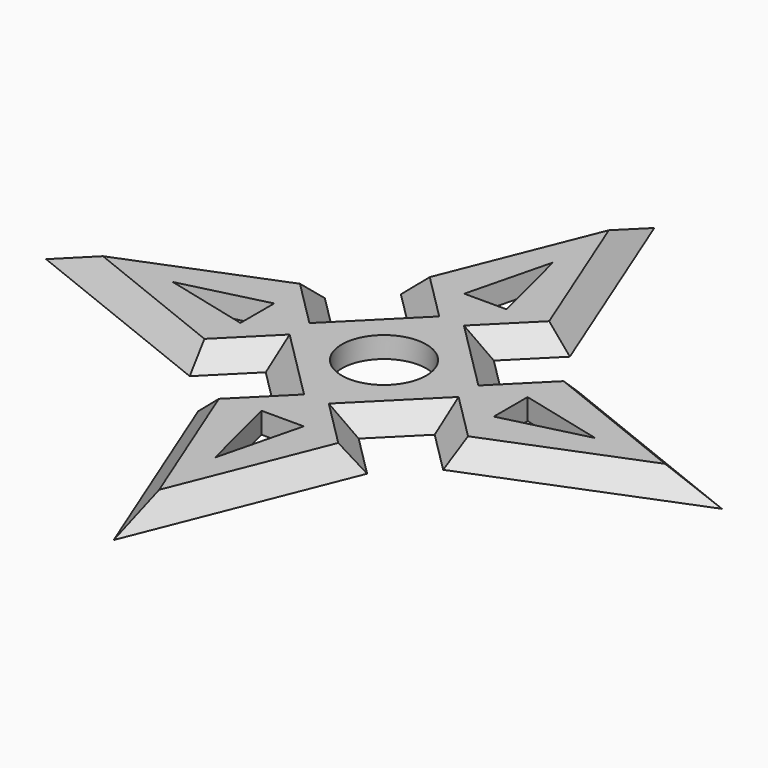
from build123d import *

# Parameters (mm, degrees)
F0_R     = 6.35
F1_DEPTH = 3.175
F2_SIZE  = 3.17499


# Not quite as in the source:
# - a fillet or chamfer is up to 0.001 mm smaller than in the source, because OpenCascade refuses the exact size


with BuildPart() as f1:
    # F0 (on Top) → F1 (new body)
    with BuildSketch(Plane.XY):
        Polygon((6.35, -12.6999929847), (-6.35, -12.6999929847), (-12.6999929847, -19.0499859695), (0, -50.7999929847), (12.6999929847, -19.0499859695), align=None)
        Polygon((-3.175, -19.0499929847), (3.175, -19.0499929847), (0, -31.7499929847), align=None, mode=Mode.SUBTRACT)
        Polygon((19.0499859695, 12.6999929847), (12.6999929847, 6.35), (12.6999929847, -6.35), (19.0499859695, -12.6999929847), (50.7999929847, 0), align=None)
        Polygon((19.0499929847, -3.175), (19.0499929847, 3.175), (31.7499929847, 0), align=None, mode=Mode.SUBTRACT)
        Polygon((-6.35, 12.6999929847), (-12.6999929847, 6.35), (-12.6999929847, -6.35), (-6.35, -12.6999929847), (6.35, -12.6999929847), (12.6999929847, -6.35), (12.6999929847, 6.35), (6.35, 12.6999929847), align=None)
        Circle(F0_R, mode=Mode.SUBTRACT)
        Polygon((-12.6999929847, -6.35), (-12.6999929847, 6.35), (-19.0499859695, 12.6999929847), (-50.7999929847, 0), (-19.0499859695, -12.6999929847), align=None)
        Polygon((-19.0499929847, 3.175), (-19.0499929847, -3.175), (-31.7499929847, 0), align=None, mode=Mode.SUBTRACT)
        Polygon((-12.6999929847, 19.0499859695), (-6.35, 12.6999929847), (6.35, 12.6999929847), (12.6999929847, 19.0499859695), (0, 50.7999929847), align=None)
        Polygon((3.175, 19.0499929847), (-3.175, 19.0499929847), (0, 31.7499929847), align=None, mode=Mode.SUBTRACT)
    extrude(amount=F1_DEPTH)

    # F2 (size 3.175 in the source; OpenCascade refuses exactly that, so slightly less here)
    f2_edges = [f1.edges().sort_by_distance(p)[0] for p in [
        (6.349996, -34.924989, 3.175),
        (-6.349996, -34.924989, 3.175),
        (-9.524996, -15.874989, 3.175),
        (9.524996, -15.874989, 3.175),
        (34.924989, -6.349996, 3.175),
        (15.874989, -9.524996, 3.175),
        (34.924989, 6.349996, 3.175),
        (15.874989, 9.524996, 3.175),
        (9.524996, -9.524996, 3.175),
        (-9.524996, -9.524996, 3.175),
        (-15.874989, -9.524996, 3.175),
        (-34.924989, -6.349996, 3.175),
        (-34.924989, 6.349996, 3.175),
        (-15.874989, 9.524996, 3.175),
        (-9.524996, 9.524996, 3.175),
        (9.524996, 9.524996, 3.175),
        (-9.524996, 15.874989, 3.175),
        (-6.349996, 34.924989, 3.175),
        (6.349996, 34.924989, 3.175),
        (9.524996, 15.874989, 3.175),
    ]]
    chamfer(f2_edges, length=F2_SIZE)


solid = f1.part
